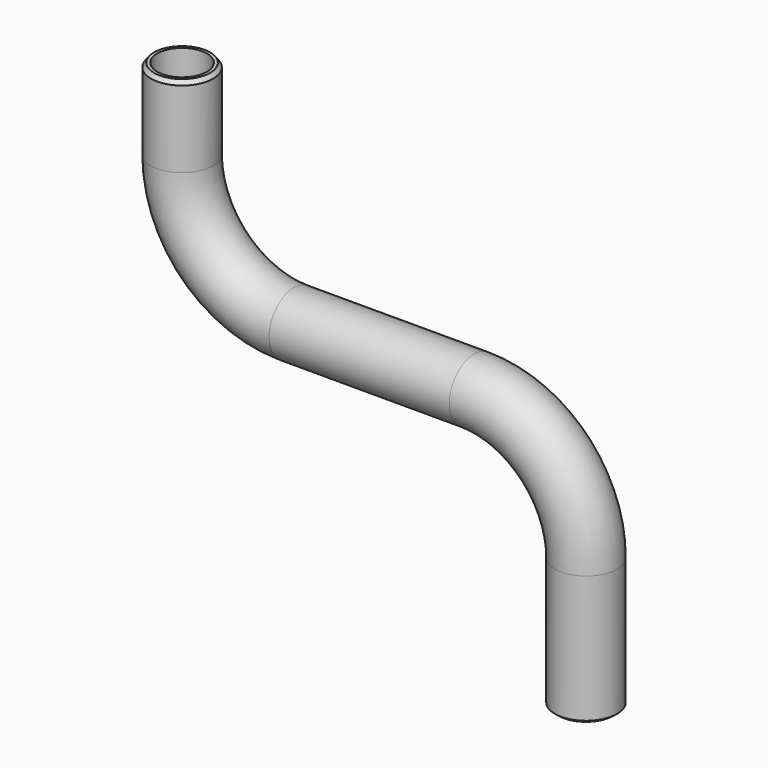
from build123d import *

# Parameters (mm, degrees)
F0_R        = 5
F0_R_2      = 4
F3_C1_SIZE2 = 0.6516126864
F3_C1_SIZE  = 0.5
F3_C2_SIZE2 = 0.5
F3_C2_SIZE  = 0.6516126864


with BuildPart() as f2:
    # F2: sweep along a path in F1
    with BuildLine(Plane.XZ) as f2_path:
        Line((0, 0), (0, 21))
        ThreePointArc((0, 21), (-5.2720779386, 33.7279220614), (-18, 39))
        Line((-18, 39), (-47, 39))
        ThreePointArc((-47, 39), (-59.7279220614, 44.2720779386), (-65, 57))
        Line((-65, 57), (-65, 70))
    # F0 (on Top) → F2 (sweep)
    with BuildSketch(Plane.XY):
        Circle(F0_R)
        Circle(F0_R_2, mode=Mode.SUBTRACT)
    sweep(path=f2_path.line)

    # F3: chamfer of 0.5 x 0.6516126864 on 2 edges, made by hand

    # F3_c1
    f3_c1_edges = [f2.edges().sort_by_distance(p)[0] for p in [
        (-5, 0, 0),
    ]]
    f3_c1_side = f2.faces().sort_by_distance((-5, 0, 0.01))[0]
    chamfer(f3_c1_edges, length=F3_C1_SIZE, length2=F3_C1_SIZE2, reference=f3_c1_side)

    # F3_c2
    f3_c2_edges = [f2.edges().sort_by_distance(p)[0] for p in [
        (-70, 0, 70),
    ]]
    f3_c2_side = f2.faces().sort_by_distance((-70, 0, 69.99))[0]
    chamfer(f3_c2_edges, length=F3_C2_SIZE, length2=F3_C2_SIZE2, reference=f3_c2_side)


solid = f2.part
